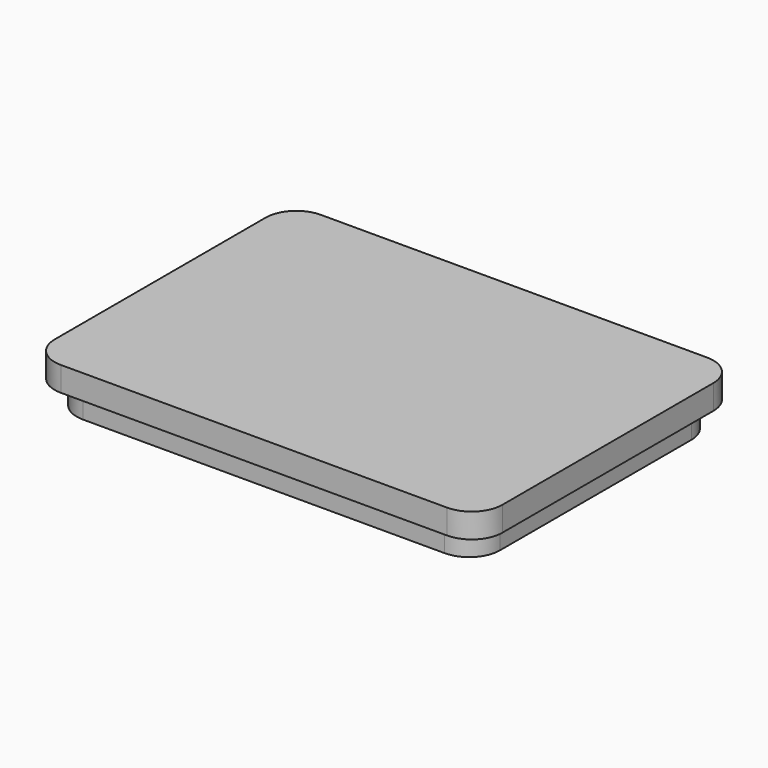
from build123d import *

# Parameters (mm, degrees)
F1_DEPTH = 8
F2_DEPTH = 8
F3_DEPTH = 4


with BuildPart() as f1:
    # F0 (on Top) → F1 (new body)
    with BuildSketch(Plane.XY):
        with BuildLine():
            Line((31.5, 26.5), (-31.5, 26.5))
            ThreePointArc((-31.5, 26.5), (-35.0355339059, 25.0355339059), (-36.5, 21.5))
            Line((-36.5, 21.5), (-36.5, -21.5))
            ThreePointArc((-36.5, -21.5), (-35.0355339059, -25.0355339059), (-31.5, -26.5))
            Line((-31.5, -26.5), (31.5, -26.5))
            ThreePointArc((31.5, -26.5), (35.0355339059, -25.0355339059), (36.5, -21.5))
            Line((36.5, -21.5), (36.5, 21.5))
            ThreePointArc((36.5, 21.5), (35.0355339059, 25.0355339059), (31.5, 26.5))
        make_face()
        with BuildLine():
            ThreePointArc((-34.5, 19.5), (-33.0355339059, 23.0355339059), (-29.5, 24.5))
            Line((-29.5, 24.5), (29.5, 24.5))
            ThreePointArc((29.5, 24.5), (33.0355339059, 23.0355339059), (34.5, 19.5))
            Line((34.5, 19.5), (34.5, -19.5))
            ThreePointArc((34.5, -19.5), (33.0355339059, -23.0355339059), (29.5, -24.5))
            Line((29.5, -24.5), (-29.5, -24.5))
            ThreePointArc((-29.5, -24.5), (-33.0355339059, -23.0355339059), (-34.5, -19.5))
            Line((-34.5, -19.5), (-34.5, 19.5))
        make_face(mode=Mode.SUBTRACT)
        with BuildLine():
            Line((29.5, 24.5), (-29.5, 24.5))
            ThreePointArc((-29.5, 24.5), (-33.0355339059, 23.0355339059), (-34.5, 19.5))
            Line((-34.5, 19.5), (-34.5, -19.5))
            ThreePointArc((-34.5, -19.5), (-33.0355339059, -23.0355339059), (-29.5, -24.5))
            Line((-29.5, -24.5), (29.5, -24.5))
            ThreePointArc((29.5, -24.5), (33.0355339059, -23.0355339059), (34.5, -19.5))
            Line((34.5, -19.5), (34.5, 19.5))
            ThreePointArc((34.5, 19.5), (33.0355339059, 23.0355339059), (29.5, 24.5))
        make_face()
    extrude(amount=F1_DEPTH)

    # F0 (on Top) → F2 (join)
    with BuildSketch(Plane.XY):
        with BuildLine():
            Line((31.5, 26.5), (-31.5, 26.5))
            ThreePointArc((-31.5, 26.5), (-35.0355339059, 25.0355339059), (-36.5, 21.5))
            Line((-36.5, 21.5), (-36.5, -21.5))
            ThreePointArc((-36.5, -21.5), (-35.0355339059, -25.0355339059), (-31.5, -26.5))
            Line((-31.5, -26.5), (31.5, -26.5))
            ThreePointArc((31.5, -26.5), (35.0355339059, -25.0355339059), (36.5, -21.5))
            Line((36.5, -21.5), (36.5, 21.5))
            ThreePointArc((36.5, 21.5), (35.0355339059, 25.0355339059), (31.5, 26.5))
        make_face()
        with BuildLine():
            ThreePointArc((-34.5, 19.5), (-33.0355339059, 23.0355339059), (-29.5, 24.5))
            Line((-29.5, 24.5), (29.5, 24.5))
            ThreePointArc((29.5, 24.5), (33.0355339059, 23.0355339059), (34.5, 19.5))
            Line((34.5, 19.5), (34.5, -19.5))
            ThreePointArc((34.5, -19.5), (33.0355339059, -23.0355339059), (29.5, -24.5))
            Line((29.5, -24.5), (-29.5, -24.5))
            ThreePointArc((-29.5, -24.5), (-33.0355339059, -23.0355339059), (-34.5, -19.5))
            Line((-34.5, -19.5), (-34.5, 19.5))
        make_face(mode=Mode.SUBTRACT)
    extrude(amount=F2_DEPTH)

    # F0 (on Top) → F3 (cut)
    with BuildSketch(Plane.XY):
        with BuildLine():
            Line((31.5, 26.5), (-31.5, 26.5))
            ThreePointArc((-31.5, 26.5), (-35.0355339059, 25.0355339059), (-36.5, 21.5))
            Line((-36.5, 21.5), (-36.5, -21.5))
            ThreePointArc((-36.5, -21.5), (-35.0355339059, -25.0355339059), (-31.5, -26.5))
            Line((-31.5, -26.5), (31.5, -26.5))
            ThreePointArc((31.5, -26.5), (35.0355339059, -25.0355339059), (36.5, -21.5))
            Line((36.5, -21.5), (36.5, 21.5))
            ThreePointArc((36.5, 21.5), (35.0355339059, 25.0355339059), (31.5, 26.5))
        make_face()
        with BuildLine():
            ThreePointArc((-34.5, 19.5), (-33.0355339059, 23.0355339059), (-29.5, 24.5))
            Line((-29.5, 24.5), (29.5, 24.5))
            ThreePointArc((29.5, 24.5), (33.0355339059, 23.0355339059), (34.5, 19.5))
            Line((34.5, 19.5), (34.5, -19.5))
            ThreePointArc((34.5, -19.5), (33.0355339059, -23.0355339059), (29.5, -24.5))
            Line((29.5, -24.5), (-29.5, -24.5))
            ThreePointArc((-29.5, -24.5), (-33.0355339059, -23.0355339059), (-34.5, -19.5))
            Line((-34.5, -19.5), (-34.5, 19.5))
        make_face(mode=Mode.SUBTRACT)
    extrude(amount=F3_DEPTH, mode=Mode.SUBTRACT)


solid = f1.part
